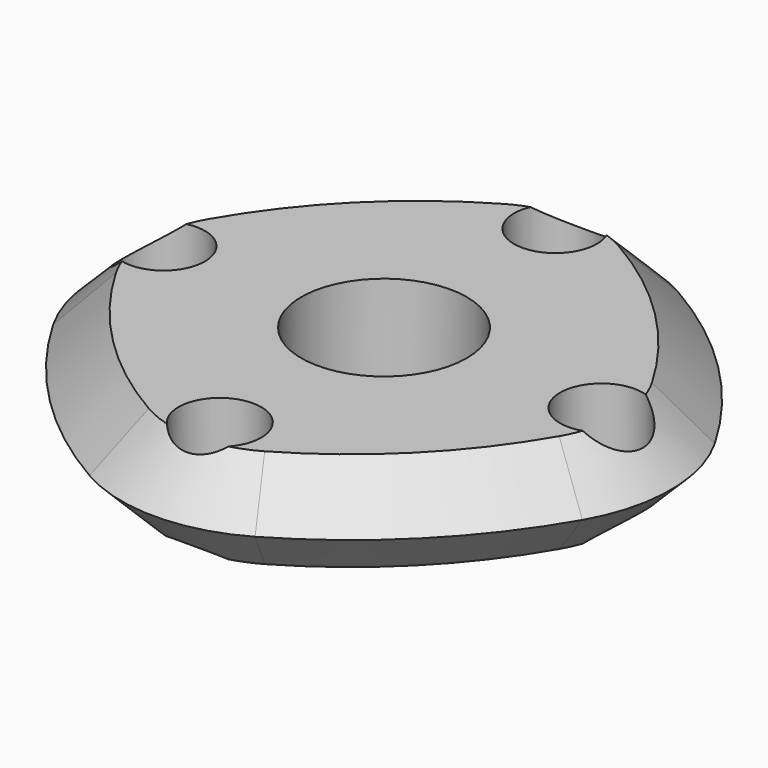
from build123d import *

# Parameters (mm, degrees)
F0_W         = 50.8
F0_H         = 50.8
F0_R         = 6.35
F1_DEPTH     = 7.62
F2_T1_DEPTH  = 198.12
F4_D         = 6.35
F5_R         = 12.7
F6_T2_ANGLE  = 29.9999999999
F6_T4_ANGLE  = 29.9999999999
F6_T6_ANGLE  = 60.000000035
F6_T8_ANGLE  = 60.000000035
F6_T10_ANGLE = 29.9999999999
F6_T12_ANGLE = 60.000000035
F6_T14_ANGLE = 29.9999999999
F6_T16_ANGLE = 60.000000035
F6_T18_ANGLE = 29.9999999999
F6_T20_ANGLE = 60.000000035
F6_T22_ANGLE = 60.000000035
F6_T24_ANGLE = 29.9999999999
F6_T26_ANGLE = 60.000000035
F6_T28_ANGLE = 29.9999999999
F6_T30_ANGLE = 60.000000035
F6_T32_ANGLE = 29.9999999999


# Not quite as in the source:
# - a fillet or chamfer that OpenCascade refuses, or shapes differently, is made with other operations: its cross-section is extruded or revolved along the edge and cut away or added


with BuildPart() as f1:
    # F0 (on Top) → F1 (new body)
    with BuildSketch(Plane.XY):
        Rectangle(F0_W, F0_H)
        Circle(F0_R, mode=Mode.SUBTRACT)
    extrude(amount=F1_DEPTH)

    # F2: fillet of radius 38.1 on 4 edges, made by hand

    # F2_s2 → F2_t1 (cut)
    with BuildSketch(Plane.XY.offset(-95.25)):
        with BuildLine():
            ThreePointArc((25.4, 12.7), (14.2407683632, -14.2407683632), (-12.7, -25.4))
            Line((-12.7, -25.4), (25.4, -25.4))
            Line((25.4, -25.4), (25.4, 12.7))
        make_face()
        with BuildLine():
            ThreePointArc((-25.4, 12.7), (-14.2407683632, -14.2407683632), (12.7, -25.4))
            Line((12.7, -25.4), (-25.4, -25.4))
            Line((-25.4, -25.4), (-25.4, 12.7))
        make_face()
        with BuildLine():
            ThreePointArc((12.7, 25.4), (-14.2407683632, 14.2407683632), (-25.4, -12.7))
            Line((-25.4, -12.7), (-25.4, 25.4))
            Line((-25.4, 25.4), (12.7, 25.4))
        make_face()
        with BuildLine():
            ThreePointArc((25.4, -12.7), (14.2407683632, 14.2407683632), (-12.7, 25.4))
            Line((-12.7, 25.4), (25.4, 25.4))
            Line((25.4, 25.4), (25.4, -12.7))
        make_face()
    extrude(amount=F2_T1_DEPTH, mode=Mode.SUBTRACT)

    # F4 (through all)
    with Locations(Plane(origin=(0, 0, 0), x_dir=(1, 0, 0), z_dir=(0, 0, -1))):
        with Locations((0, -16.4350587875), (-16.9112086296, 0), (0, 15.7412625849), (16.6794583201, 0)):
            Hole(F4_D / 2)

    # F5
    f5_edges = [f1.edges().sort_by_distance(p)[0] for p in [
        (0, -23.221024, 3.81),
        (23.221024, 0, 3.81),
        (-23.221024, 0, 3.81),
        (0, 23.221024, 3.81),
    ]]
    fillet(f5_edges, radius=F5_R)

    # F6: chamfer of 3.81 on 2 edges, made by hand

    # F6_s1 → F6_t2 (revolve, cut)
    with BuildSketch(Plane(origin=(2.324261314, 4.025738686, 0), x_dir=(0, 0, 1), z_dir=(0.5, 0.8660254038, 0))):
        Polygon((3.81, 20.7514773719), (7.62, 16.9414773719), (7.62, 20.7514773719), align=None)
    revolve(axis=Axis((-12.7, 12.7, 7.62), (0, 0, -1)), revolution_arc=F6_T2_ANGLE, mode=Mode.SUBTRACT)

    # F6_s3 → F6_t4 (revolve, cut)
    with BuildSketch(Plane(origin=(2.324261314, 4.025738686, 0), x_dir=(0, 0, 1), z_dir=(0.5, 0.8660254038, 0))):
        Polygon((0, 16.9414773719), (3.81, 20.7514773719), (0, 20.7514773719), align=None)
    revolve(axis=Axis((-12.7, 12.7, 0), (0, 0, -1)), revolution_arc=F6_T4_ANGLE, mode=Mode.SUBTRACT)

    # F6_s5 → F6_t6 (revolve, cut)
    with BuildSketch(Plane(origin=(2.324261317, -4.0257386892, 0), x_dir=(0, 0, 1), z_dir=(-0.5000000002, 0.8660254037, 0))):
        Polygon((0, 16.941477371), (3.81, 20.7514773707), (0, 20.751477371), align=None)
    revolve(axis=Axis((9.2970452639, 1.5e-09, 0), (0, 0, -1)), revolution_arc=F6_T6_ANGLE, mode=Mode.SUBTRACT)

    # F6_s7 → F6_t8 (revolve, cut)
    with BuildSketch(Plane(origin=(4.0257386892, -2.324261317, 0), x_dir=(0, 0, 1), z_dir=(-0.8660254037, 0.5000000002, 0))):
        Polygon((0, -16.941477371), (3.81, -20.7514773707), (0, -20.751477371), align=None)
    revolve(axis=Axis((-1.5e-09, -9.2970452639, 0), (0, 0, 1)), revolution_arc=F6_T8_ANGLE, mode=Mode.SUBTRACT)

    # F6_s9 → F6_t10 (revolve, cut)
    with BuildSketch(Plane(origin=(4.025738686, -2.324261314, 0), x_dir=(0, 0, 1), z_dir=(0.8660254038, -0.5, 0))):
        Polygon((0, 16.9414773719), (3.81, 20.7514773719), (0, 20.7514773719), align=None)
    revolve(axis=Axis((12.7, 12.7, 0), (0, 0, -1)), revolution_arc=F6_T10_ANGLE, mode=Mode.SUBTRACT)

    # F6_s11 → F6_t12 (revolve, cut)
    with BuildSketch(Plane(origin=(-2.324261317, -4.0257386892, 0), x_dir=(0, 0, 1), z_dir=(0.5000000002, 0.8660254037, 0))):
        Polygon((0, -16.941477371), (3.81, -20.7514773707), (0, -20.751477371), align=None)
    revolve(axis=Axis((-9.2970452639, 1.5e-09, 0), (0, 0, 1)), revolution_arc=F6_T12_ANGLE, mode=Mode.SUBTRACT)

    # F6_s13 → F6_t14 (revolve, cut)
    with BuildSketch(Plane(origin=(-2.324261314, -4.025738686, 0), x_dir=(0, 0, 1), z_dir=(-0.5, -0.8660254038, 0))):
        Polygon((0, 16.9414773719), (3.81, 20.7514773719), (0, 20.7514773719), align=None)
    revolve(axis=Axis((12.7, -12.7, 0), (0, 0, -1)), revolution_arc=F6_T14_ANGLE, mode=Mode.SUBTRACT)

    # F6_s15 → F6_t16 (revolve, cut)
    with BuildSketch(Plane(origin=(4.0257386892, 2.324261317, 0), x_dir=(0, 0, 1), z_dir=(-0.8660254037, -0.5000000002, 0))):
        Polygon((0, 16.941477371), (3.81, 20.7514773707), (0, 20.751477371), align=None)
    revolve(axis=Axis((-1.5e-09, 9.2970452639, 0), (0, 0, -1)), revolution_arc=F6_T16_ANGLE, mode=Mode.SUBTRACT)

    # F6_s17 → F6_t18 (revolve, cut)
    with BuildSketch(Plane(origin=(-4.025738686, 2.324261314, 0), x_dir=(0, 0, 1), z_dir=(-0.8660254038, 0.5, 0))):
        Polygon((0, 16.9414773719), (3.81, 20.7514773719), (0, 20.7514773719), align=None)
    revolve(axis=Axis((-12.7, -12.7, 0), (0, 0, -1)), revolution_arc=F6_T18_ANGLE, mode=Mode.SUBTRACT)

    # F6_s19 → F6_t20 (revolve, cut)
    with BuildSketch(Plane(origin=(2.324261317, -4.0257386892, 0), x_dir=(0, 0, 1), z_dir=(-0.5000000002, 0.8660254037, 0))):
        Polygon((3.81, 20.7514773707), (7.62, 16.941477371), (7.62, 20.751477371), align=None)
    revolve(axis=Axis((9.2970452639, 1.5e-09, 7.62), (0, 0, -1)), revolution_arc=F6_T20_ANGLE, mode=Mode.SUBTRACT)

    # F6_s21 → F6_t22 (revolve, cut)
    with BuildSketch(Plane(origin=(4.0257386892, -2.324261317, 0), x_dir=(0, 0, 1), z_dir=(-0.8660254037, 0.5000000002, 0))):
        Polygon((3.81, -20.7514773707), (7.62, -16.941477371), (7.62, -20.751477371), align=None)
    revolve(axis=Axis((-1.5e-09, -9.2970452639, 7.62), (0, 0, 1)), revolution_arc=F6_T22_ANGLE, mode=Mode.SUBTRACT)

    # F6_s23 → F6_t24 (revolve, cut)
    with BuildSketch(Plane(origin=(4.025738686, -2.324261314, 0), x_dir=(0, 0, 1), z_dir=(0.8660254038, -0.5, 0))):
        Polygon((3.81, 20.7514773719), (7.62, 16.9414773719), (7.62, 20.7514773719), align=None)
    revolve(axis=Axis((12.7, 12.7, 7.62), (0, 0, -1)), revolution_arc=F6_T24_ANGLE, mode=Mode.SUBTRACT)

    # F6_s25 → F6_t26 (revolve, cut)
    with BuildSketch(Plane(origin=(-2.324261317, -4.0257386892, 0), x_dir=(0, 0, 1), z_dir=(0.5000000002, 0.8660254037, 0))):
        Polygon((3.81, -20.7514773707), (7.62, -16.941477371), (7.62, -20.751477371), align=None)
    revolve(axis=Axis((-9.2970452639, 1.5e-09, 7.62), (0, 0, 1)), revolution_arc=F6_T26_ANGLE, mode=Mode.SUBTRACT)

    # F6_s27 → F6_t28 (revolve, cut)
    with BuildSketch(Plane(origin=(-2.324261314, -4.025738686, 0), x_dir=(0, 0, 1), z_dir=(-0.5, -0.8660254038, 0))):
        Polygon((3.81, 20.7514773719), (7.62, 16.9414773719), (7.62, 20.7514773719), align=None)
    revolve(axis=Axis((12.7, -12.7, 7.62), (0, 0, -1)), revolution_arc=F6_T28_ANGLE, mode=Mode.SUBTRACT)

    # F6_s29 → F6_t30 (revolve, cut)
    with BuildSketch(Plane(origin=(4.0257386892, 2.324261317, 0), x_dir=(0, 0, 1), z_dir=(-0.8660254037, -0.5000000002, 0))):
        Polygon((3.81, 20.7514773707), (7.62, 16.941477371), (7.62, 20.751477371), align=None)
    revolve(axis=Axis((-1.5e-09, 9.2970452639, 7.62), (0, 0, -1)), revolution_arc=F6_T30_ANGLE, mode=Mode.SUBTRACT)

    # F6_s31 → F6_t32 (revolve, cut)
    with BuildSketch(Plane(origin=(-4.025738686, 2.324261314, 0), x_dir=(0, 0, 1), z_dir=(-0.8660254038, 0.5, 0))):
        Polygon((3.81, 20.7514773719), (7.62, 16.9414773719), (7.62, 20.7514773719), align=None)
    revolve(axis=Axis((-12.7, -12.7, 7.62), (0, 0, -1)), revolution_arc=F6_T32_ANGLE, mode=Mode.SUBTRACT)


solid = f1.part
